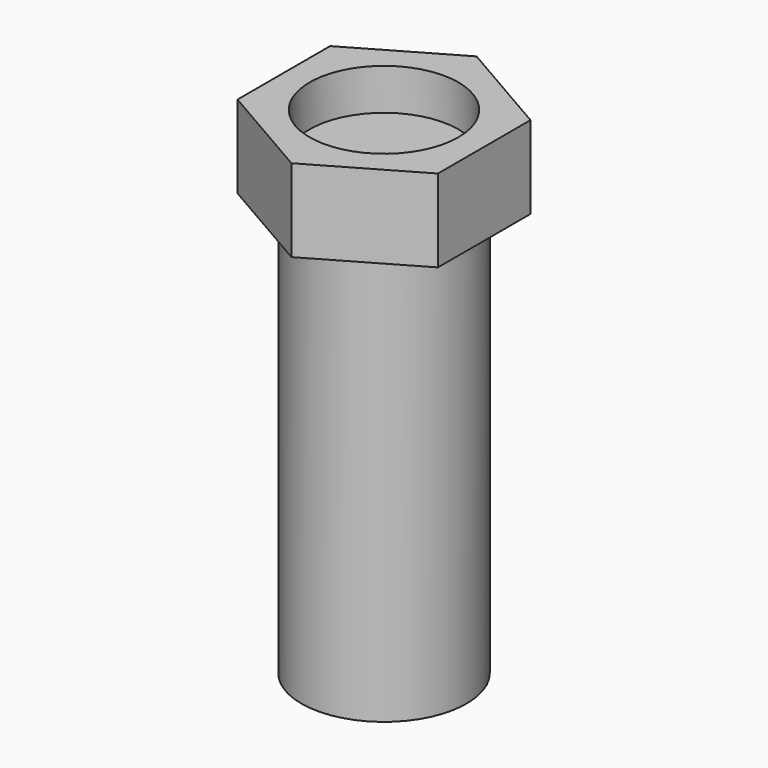
from build123d import *

# Parameters (mm, degrees)
F0_W     = 0.25
F0_H     = 1.25
F2_R     = 0.25
F3_DEPTH = 0.25
F4_R     = 0.225
F5_DEPTH = 0.125


with BuildPart() as f1:
    # F0 (on Front) → F1 (revolve)
    with BuildSketch(Plane.XZ):
        with Locations((-0.125, 0.625)):
            Rectangle(F0_W, F0_H)
    revolve(axis=Axis((0, 0, 0.625), (0, 0, 1)))

    # F2 (on face) → F3 (join)
    with BuildSketch(Plane.XY.offset(1.25)):
        Polygon((0.3031088913, 0.175), (0, 0.35), (-0.3031088913, 0.175), (-0.3031088913, -0.175), (0, -0.35), (0.3031088913, -0.175), align=None)
        Circle(F2_R, mode=Mode.SUBTRACT)
        Circle(F2_R)
    extrude(amount=F3_DEPTH)

    # F4 (on face) → F5 (cut)
    with BuildSketch(Plane.XY.offset(1.5)):
        Circle(F4_R)
    extrude(amount=-F5_DEPTH, mode=Mode.SUBTRACT)


solid = f1.part
